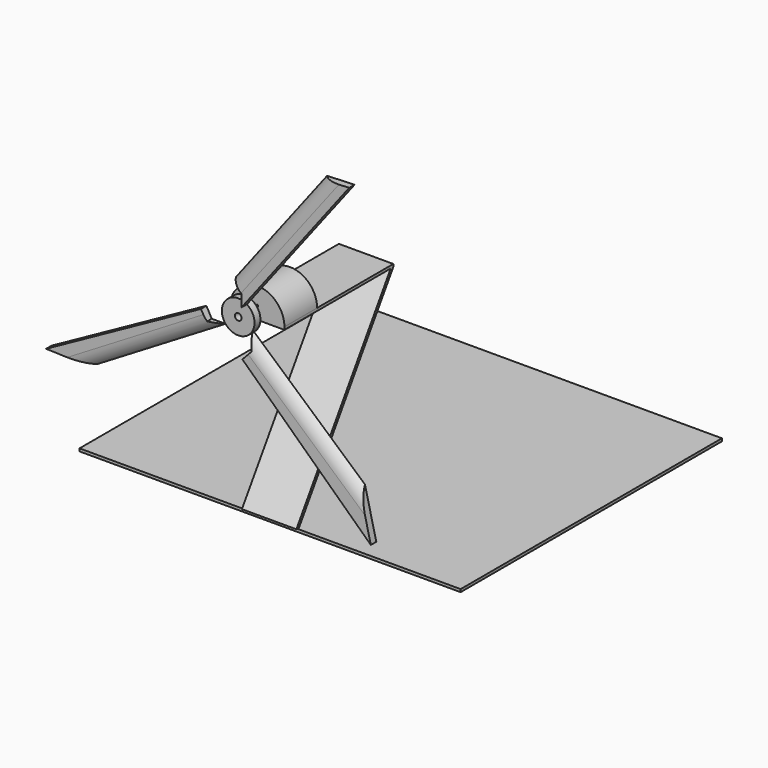
from build123d import *

# Parameters (mm, degrees)
F0_W           = 140
F0_H           = 120
F1_DEPTH       = 1
F4_DEPTH       = 10
F5_W           = 20
F5_H           = 50
F6_DEPTH       = 1
F8_DEPTH       = 15
F9_R           = 0.4
F10_DEPTH      = 4
F11_R          = 1.2398278846
F12_DEPTH      = 2
F13_R          = 6
F13_R_2        = 1.2398278846
F14_DEPTH      = 2.7
F16_DEPTH      = 2.5
F17_T1_DEPTH   = 79.366985862
F17_2_T1_DEPTH = 79.366985862
F17_3_T1_DEPTH = 79.366985862


# Not quite as in the source:
# - a fillet or chamfer that OpenCascade refuses, or shapes differently, is made with other operations: its cross-section is extruded or revolved along the edge and cut away or added


with BuildPart() as f1:
    # F0 (on Top) → F1 (new body)
    with BuildSketch(Plane.XY):
        with Locations((70, 60)):
            Rectangle(F0_W, F0_H)
    extrude(amount=F1_DEPTH)


with BuildPart() as f4:
    # F3 (on offset) → F4 (new body, symmetric)
    with BuildSketch(Plane.YZ.offset(70)):
        Polygon((-0.4200659473, 1.0160847374), (0.7722973455, 1.0160847374), (43.7408067697, 67.1817869472), (44.0944994946, 67.7264259822), (42.9021362018, 67.7264259822), align=None)
    extrude(amount=F4_DEPTH, both=True)

    # F5 (on face) → F6 (join)
    with BuildSketch(Plane.XY.offset(67.7264259822)):
        with Locations((70, 19.0944994946)):
            Rectangle(F5_W, F5_H)
    extrude(amount=F6_DEPTH)

    # F7 (on face) → F8 (join)
    with BuildSketch(Plane.XZ.offset(5.9055005054)):
        with BuildLine():
            Line((60, 68.7264259822), (80, 68.7264259822))
            ThreePointArc((80, 68.7264259822), (70, 78.7264259822), (60, 68.7264259822))
        make_face()
    extrude(amount=-F8_DEPTH)

    # F9 (on face) → F10 (join)
    with BuildSketch(Plane.XZ.offset(5.9055005054)):
        with Locations((69.9867457151, 72.2166821361)):
            Circle(F9_R)
    extrude(amount=F10_DEPTH)

    # F11 (on face) → F12 (join)
    with BuildSketch(Plane.XZ.offset(9.9055005054)):
        with Locations((69.9867457151, 72.2166821361)):
            Circle(F11_R)
    extrude(amount=F12_DEPTH)


with BuildPart() as f14:
    # F13 (on face) → F14 (new body)
    with BuildSketch(Plane.XZ.offset(11.9055005054)):
        with Locations((69.9867457151, 72.2166821361)):
            Circle(F13_R)
        with Locations((69.9867457151, 72.2166821361)):
            Circle(F13_R_2, mode=Mode.SUBTRACT)
    extrude(amount=F14_DEPTH)


with BuildPart() as f16:
    # F15 (on face) → F16 (new body)
    with BuildSketch(Plane.XZ.offset(14.6055005054)):
        Polygon((116.5578424183, 33.1474154847), (75.4019039591, 69.6328746368), (76.7731679631, 64.0930237523), (73.5093057156, 60.6463849545), (120.7056262574, 15.9529030212), align=None)
    extrude(amount=F16_DEPTH)

    # F17: fillet of radius 6 on 1 edges, made by hand

    # F17_s2 → F17_t1 (cut)
    with BuildSketch(Plane(origin=(57.9277089102, 0, -51.3539269506), x_dir=(0, 1, 0), z_dir=(-0.7482897902, 0, 0.6633719846))):
        with BuildLine():
            ThreePointArc((-14.6055005054, -102.1250798215), (-16.4440396314, -99.9902954366), (-17.1055005054, -97.2516826491))
            Line((-17.1055005054, -97.2516826491), (-17.1055005054, -102.1250798215))
            Line((-17.1055005054, -102.1250798215), (-14.6055005054, -102.1250798215))
        make_face()
    extrude(amount=F17_T1_DEPTH, mode=Mode.SUBTRACT)


with BuildPart() as f16b:
    # F15 (on face) → F16, piece 2 (new body)
    with BuildSketch(Plane.XZ.offset(14.6055005054)):
        Polygon((73.1090417788, 81.7856717816), (73.1698371178, 77.3027345465), (112.7452876158, 128.8661296819), (102.6347893563, 128.4564783105), (69.1478697041, 84.825913196), align=None)
    extrude(amount=F16_DEPTH)

    # F17#2: fillet of radius 6 on 1 edges, made by hand

    # F17_2_s2 → F17_2_t1 (cut)
    with BuildSketch(Plane(origin=(107.5084414965, 0, 140.0742172108), x_dir=(0, 1, 0), z_dir=(-0.6088530846, 0, -0.7932830021))):
        with BuildLine():
            ThreePointArc((-14.6055005054, 3.2073107645), (-16.4440396314, 5.3420951494), (-17.1055005054, 8.0807079369))
            Line((-17.1055005054, 8.0807079369), (-17.1055005054, 3.2073107645))
            Line((-17.1055005054, 3.2073107645), (-14.6055005054, 3.2073107645))
        make_face()
    extrude(amount=F17_2_T1_DEPTH, mode=Mode.SUBTRACT)


with BuildPart() as f16c:
    # F15 (on face) → F16, piece 3 (new body)
    with BuildSketch(Plane.XZ.offset(14.6055005054)):
        Polygon((18.1934121118, 40.0880810557), (65.3174607263, 68.4486882808), (60.2683858732, 68.4486882808), (58.3051553434, 72.0047285657), (1.4012531219, 40.5890332532), align=None)
    extrude(amount=F16_DEPTH)

    # F17#3: fillet of radius 6 on 1 edges, made by hand

    # F17_3_s2 → F17_3_t1 (cut)
    with BuildSketch(Plane(origin=(20.6282983072, 0, 12.4147029641), x_dir=(0, 1, 0), z_dir=(0.8568008839, 0, 0.5156474041))):
        with BuildLine():
            ThreePointArc((-14.6055005054, 24.9661175553), (-16.4440396314, 27.1009019401), (-17.1055005054, 29.8395147277))
            Line((-17.1055005054, 29.8395147277), (-17.1055005054, 24.9661175553))
            Line((-17.1055005054, 24.9661175553), (-14.6055005054, 24.9661175553))
        make_face()
    extrude(amount=F17_3_T1_DEPTH, mode=Mode.SUBTRACT)


solid = Compound([f1.part, f4.part, f14.part, f16.part, f16b.part, f16c.part])
